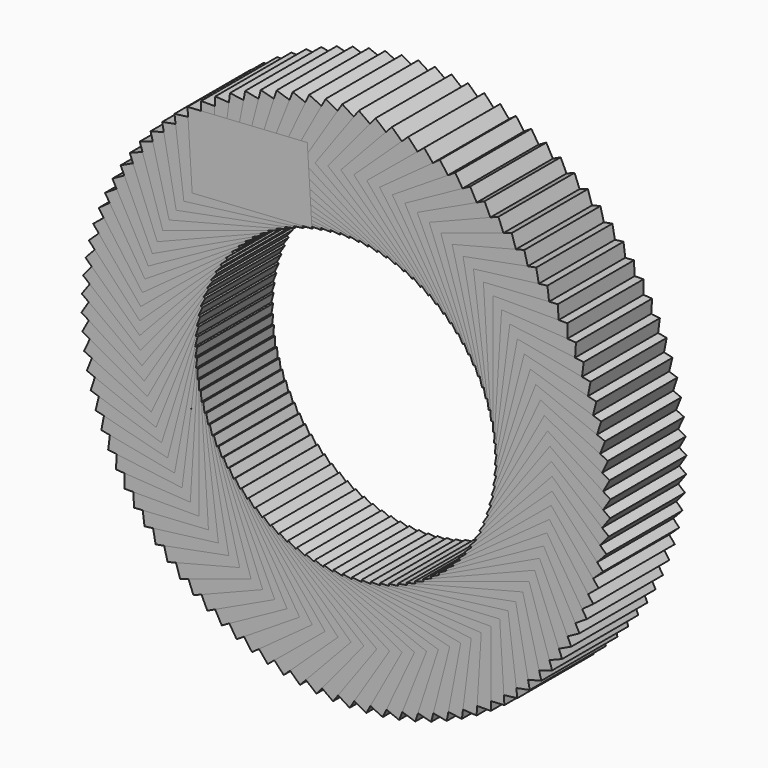
from build123d import *

# Parameters (mm, degrees)
F0_W            = 95.955953002
F0_H            = 59.5492273569
F1_DEPTH        = 76.0588273406
F1_COPIES_COUNT = 100


# Not quite as in the source:
# - a feature of the source that left no trace in its solid (it failed there, or was rolled back) is left out
# - a pattern or mirror of a feature is missing from the dataset's text; its kind, count and spacing are read off the source's solid
# - the program builds the solid bodies; features that only make, move or delete a surface that nothing else refers to are left out


with BuildPart() as f1:
    # F0 (on Front) → F1 (new body)
    with BuildSketch(Plane.XZ):
        with Locations((-90.7992497087, 42.9625064135)):
            Rectangle(F0_W, F0_H)
    extrude(amount=F1_DEPTH)


with BuildPart() as f1_copies_1:
    # F1_copies: instance of F1
    add(f1.part.rotate(Axis((-23.007184, 0, -104.193181), (0, 1, 0)), 1 * 360 / F1_COPIES_COUNT))


with BuildPart() as f1_copies_2:
    # F1_copies: instance of F1
    add(f1.part.rotate(Axis((-23.007184, 0, -104.193181), (0, 1, 0)), 2 * 360 / F1_COPIES_COUNT))


with BuildPart() as f1_copies_3:
    # F1_copies: instance of F1
    add(f1.part.rotate(Axis((-23.007184, 0, -104.193181), (0, 1, 0)), 3 * 360 / F1_COPIES_COUNT))


with BuildPart() as f1_copies_4:
    # F1_copies: instance of F1
    add(f1.part.rotate(Axis((-23.007184, 0, -104.193181), (0, 1, 0)), 4 * 360 / F1_COPIES_COUNT))


with BuildPart() as f1_copies_5:
    # F1_copies: instance of F1
    add(f1.part.rotate(Axis((-23.007184, 0, -104.193181), (0, 1, 0)), 5 * 360 / F1_COPIES_COUNT))


with BuildPart() as f1_copies_6:
    # F1_copies: instance of F1
    add(f1.part.rotate(Axis((-23.007184, 0, -104.193181), (0, 1, 0)), 6 * 360 / F1_COPIES_COUNT))


with BuildPart() as f1_copies_7:
    # F1_copies: instance of F1
    add(f1.part.rotate(Axis((-23.007184, 0, -104.193181), (0, 1, 0)), 7 * 360 / F1_COPIES_COUNT))


with BuildPart() as f1_copies_8:
    # F1_copies: instance of F1
    add(f1.part.rotate(Axis((-23.007184, 0, -104.193181), (0, 1, 0)), 8 * 360 / F1_COPIES_COUNT))


with BuildPart() as f1_copies_9:
    # F1_copies: instance of F1
    add(f1.part.rotate(Axis((-23.007184, 0, -104.193181), (0, 1, 0)), 9 * 360 / F1_COPIES_COUNT))


with BuildPart() as f1_copies_10:
    # F1_copies: instance of F1
    add(f1.part.rotate(Axis((-23.007184, 0, -104.193181), (0, 1, 0)), 10 * 360 / F1_COPIES_COUNT))


with BuildPart() as f1_copies_11:
    # F1_copies: instance of F1
    add(f1.part.rotate(Axis((-23.007184, 0, -104.193181), (0, 1, 0)), 11 * 360 / F1_COPIES_COUNT))


with BuildPart() as f1_copies_12:
    # F1_copies: instance of F1
    add(f1.part.rotate(Axis((-23.007184, 0, -104.193181), (0, 1, 0)), 12 * 360 / F1_COPIES_COUNT))


with BuildPart() as f1_copies_13:
    # F1_copies: instance of F1
    add(f1.part.rotate(Axis((-23.007184, 0, -104.193181), (0, 1, 0)), 13 * 360 / F1_COPIES_COUNT))


with BuildPart() as f1_copies_14:
    # F1_copies: instance of F1
    add(f1.part.rotate(Axis((-23.007184, 0, -104.193181), (0, 1, 0)), 14 * 360 / F1_COPIES_COUNT))


with BuildPart() as f1_copies_15:
    # F1_copies: instance of F1
    add(f1.part.rotate(Axis((-23.007184, 0, -104.193181), (0, 1, 0)), 15 * 360 / F1_COPIES_COUNT))


with BuildPart() as f1_copies_16:
    # F1_copies: instance of F1
    add(f1.part.rotate(Axis((-23.007184, 0, -104.193181), (0, 1, 0)), 16 * 360 / F1_COPIES_COUNT))


with BuildPart() as f1_copies_17:
    # F1_copies: instance of F1
    add(f1.part.rotate(Axis((-23.007184, 0, -104.193181), (0, 1, 0)), 17 * 360 / F1_COPIES_COUNT))


with BuildPart() as f1_copies_18:
    # F1_copies: instance of F1
    add(f1.part.rotate(Axis((-23.007184, 0, -104.193181), (0, 1, 0)), 18 * 360 / F1_COPIES_COUNT))


with BuildPart() as f1_copies_19:
    # F1_copies: instance of F1
    add(f1.part.rotate(Axis((-23.007184, 0, -104.193181), (0, 1, 0)), 19 * 360 / F1_COPIES_COUNT))


with BuildPart() as f1_copies_20:
    # F1_copies: instance of F1
    add(f1.part.rotate(Axis((-23.007184, 0, -104.193181), (0, 1, 0)), 20 * 360 / F1_COPIES_COUNT))


with BuildPart() as f1_copies_21:
    # F1_copies: instance of F1
    add(f1.part.rotate(Axis((-23.007184, 0, -104.193181), (0, 1, 0)), 21 * 360 / F1_COPIES_COUNT))


with BuildPart() as f1_copies_22:
    # F1_copies: instance of F1
    add(f1.part.rotate(Axis((-23.007184, 0, -104.193181), (0, 1, 0)), 22 * 360 / F1_COPIES_COUNT))


with BuildPart() as f1_copies_23:
    # F1_copies: instance of F1
    add(f1.part.rotate(Axis((-23.007184, 0, -104.193181), (0, 1, 0)), 23 * 360 / F1_COPIES_COUNT))


with BuildPart() as f1_copies_24:
    # F1_copies: instance of F1
    add(f1.part.rotate(Axis((-23.007184, 0, -104.193181), (0, 1, 0)), 24 * 360 / F1_COPIES_COUNT))


with BuildPart() as f1_copies_25:
    # F1_copies: instance of F1
    add(f1.part.rotate(Axis((-23.007184, 0, -104.193181), (0, 1, 0)), 25 * 360 / F1_COPIES_COUNT))


with BuildPart() as f1_copies_26:
    # F1_copies: instance of F1
    add(f1.part.rotate(Axis((-23.007184, 0, -104.193181), (0, 1, 0)), 26 * 360 / F1_COPIES_COUNT))


with BuildPart() as f1_copies_27:
    # F1_copies: instance of F1
    add(f1.part.rotate(Axis((-23.007184, 0, -104.193181), (0, 1, 0)), 27 * 360 / F1_COPIES_COUNT))


with BuildPart() as f1_copies_28:
    # F1_copies: instance of F1
    add(f1.part.rotate(Axis((-23.007184, 0, -104.193181), (0, 1, 0)), 28 * 360 / F1_COPIES_COUNT))


with BuildPart() as f1_copies_29:
    # F1_copies: instance of F1
    add(f1.part.rotate(Axis((-23.007184, 0, -104.193181), (0, 1, 0)), 29 * 360 / F1_COPIES_COUNT))


with BuildPart() as f1_copies_30:
    # F1_copies: instance of F1
    add(f1.part.rotate(Axis((-23.007184, 0, -104.193181), (0, 1, 0)), 30 * 360 / F1_COPIES_COUNT))


with BuildPart() as f1_copies_31:
    # F1_copies: instance of F1
    add(f1.part.rotate(Axis((-23.007184, 0, -104.193181), (0, 1, 0)), 31 * 360 / F1_COPIES_COUNT))


with BuildPart() as f1_copies_32:
    # F1_copies: instance of F1
    add(f1.part.rotate(Axis((-23.007184, 0, -104.193181), (0, 1, 0)), 32 * 360 / F1_COPIES_COUNT))


with BuildPart() as f1_copies_33:
    # F1_copies: instance of F1
    add(f1.part.rotate(Axis((-23.007184, 0, -104.193181), (0, 1, 0)), 33 * 360 / F1_COPIES_COUNT))


with BuildPart() as f1_copies_34:
    # F1_copies: instance of F1
    add(f1.part.rotate(Axis((-23.007184, 0, -104.193181), (0, 1, 0)), 34 * 360 / F1_COPIES_COUNT))


with BuildPart() as f1_copies_35:
    # F1_copies: instance of F1
    add(f1.part.rotate(Axis((-23.007184, 0, -104.193181), (0, 1, 0)), 35 * 360 / F1_COPIES_COUNT))


with BuildPart() as f1_copies_36:
    # F1_copies: instance of F1
    add(f1.part.rotate(Axis((-23.007184, 0, -104.193181), (0, 1, 0)), 36 * 360 / F1_COPIES_COUNT))


with BuildPart() as f1_copies_37:
    # F1_copies: instance of F1
    add(f1.part.rotate(Axis((-23.007184, 0, -104.193181), (0, 1, 0)), 37 * 360 / F1_COPIES_COUNT))


with BuildPart() as f1_copies_38:
    # F1_copies: instance of F1
    add(f1.part.rotate(Axis((-23.007184, 0, -104.193181), (0, 1, 0)), 38 * 360 / F1_COPIES_COUNT))


with BuildPart() as f1_copies_39:
    # F1_copies: instance of F1
    add(f1.part.rotate(Axis((-23.007184, 0, -104.193181), (0, 1, 0)), 39 * 360 / F1_COPIES_COUNT))


with BuildPart() as f1_copies_40:
    # F1_copies: instance of F1
    add(f1.part.rotate(Axis((-23.007184, 0, -104.193181), (0, 1, 0)), 40 * 360 / F1_COPIES_COUNT))


with BuildPart() as f1_copies_41:
    # F1_copies: instance of F1
    add(f1.part.rotate(Axis((-23.007184, 0, -104.193181), (0, 1, 0)), 41 * 360 / F1_COPIES_COUNT))


with BuildPart() as f1_copies_42:
    # F1_copies: instance of F1
    add(f1.part.rotate(Axis((-23.007184, 0, -104.193181), (0, 1, 0)), 42 * 360 / F1_COPIES_COUNT))


with BuildPart() as f1_copies_43:
    # F1_copies: instance of F1
    add(f1.part.rotate(Axis((-23.007184, 0, -104.193181), (0, 1, 0)), 43 * 360 / F1_COPIES_COUNT))


with BuildPart() as f1_copies_44:
    # F1_copies: instance of F1
    add(f1.part.rotate(Axis((-23.007184, 0, -104.193181), (0, 1, 0)), 44 * 360 / F1_COPIES_COUNT))


with BuildPart() as f1_copies_45:
    # F1_copies: instance of F1
    add(f1.part.rotate(Axis((-23.007184, 0, -104.193181), (0, 1, 0)), 45 * 360 / F1_COPIES_COUNT))


with BuildPart() as f1_copies_46:
    # F1_copies: instance of F1
    add(f1.part.rotate(Axis((-23.007184, 0, -104.193181), (0, 1, 0)), 46 * 360 / F1_COPIES_COUNT))


with BuildPart() as f1_copies_47:
    # F1_copies: instance of F1
    add(f1.part.rotate(Axis((-23.007184, 0, -104.193181), (0, 1, 0)), 47 * 360 / F1_COPIES_COUNT))


with BuildPart() as f1_copies_48:
    # F1_copies: instance of F1
    add(f1.part.rotate(Axis((-23.007184, 0, -104.193181), (0, 1, 0)), 48 * 360 / F1_COPIES_COUNT))


with BuildPart() as f1_copies_49:
    # F1_copies: instance of F1
    add(f1.part.rotate(Axis((-23.007184, 0, -104.193181), (0, 1, 0)), 49 * 360 / F1_COPIES_COUNT))


with BuildPart() as f1_copies_50:
    # F1_copies: instance of F1
    add(f1.part.rotate(Axis((-23.007184, 0, -104.193181), (0, 1, 0)), 50 * 360 / F1_COPIES_COUNT))


with BuildPart() as f1_copies_51:
    # F1_copies: instance of F1
    add(f1.part.rotate(Axis((-23.007184, 0, -104.193181), (0, 1, 0)), 51 * 360 / F1_COPIES_COUNT))


with BuildPart() as f1_copies_52:
    # F1_copies: instance of F1
    add(f1.part.rotate(Axis((-23.007184, 0, -104.193181), (0, 1, 0)), 52 * 360 / F1_COPIES_COUNT))


with BuildPart() as f1_copies_53:
    # F1_copies: instance of F1
    add(f1.part.rotate(Axis((-23.007184, 0, -104.193181), (0, 1, 0)), 53 * 360 / F1_COPIES_COUNT))


with BuildPart() as f1_copies_54:
    # F1_copies: instance of F1
    add(f1.part.rotate(Axis((-23.007184, 0, -104.193181), (0, 1, 0)), 54 * 360 / F1_COPIES_COUNT))


with BuildPart() as f1_copies_55:
    # F1_copies: instance of F1
    add(f1.part.rotate(Axis((-23.007184, 0, -104.193181), (0, 1, 0)), 55 * 360 / F1_COPIES_COUNT))


with BuildPart() as f1_copies_56:
    # F1_copies: instance of F1
    add(f1.part.rotate(Axis((-23.007184, 0, -104.193181), (0, 1, 0)), 56 * 360 / F1_COPIES_COUNT))


with BuildPart() as f1_copies_57:
    # F1_copies: instance of F1
    add(f1.part.rotate(Axis((-23.007184, 0, -104.193181), (0, 1, 0)), 57 * 360 / F1_COPIES_COUNT))


with BuildPart() as f1_copies_58:
    # F1_copies: instance of F1
    add(f1.part.rotate(Axis((-23.007184, 0, -104.193181), (0, 1, 0)), 58 * 360 / F1_COPIES_COUNT))


with BuildPart() as f1_copies_59:
    # F1_copies: instance of F1
    add(f1.part.rotate(Axis((-23.007184, 0, -104.193181), (0, 1, 0)), 59 * 360 / F1_COPIES_COUNT))


with BuildPart() as f1_copies_60:
    # F1_copies: instance of F1
    add(f1.part.rotate(Axis((-23.007184, 0, -104.193181), (0, 1, 0)), 60 * 360 / F1_COPIES_COUNT))


with BuildPart() as f1_copies_61:
    # F1_copies: instance of F1
    add(f1.part.rotate(Axis((-23.007184, 0, -104.193181), (0, 1, 0)), 61 * 360 / F1_COPIES_COUNT))


with BuildPart() as f1_copies_62:
    # F1_copies: instance of F1
    add(f1.part.rotate(Axis((-23.007184, 0, -104.193181), (0, 1, 0)), 62 * 360 / F1_COPIES_COUNT))


with BuildPart() as f1_copies_63:
    # F1_copies: instance of F1
    add(f1.part.rotate(Axis((-23.007184, 0, -104.193181), (0, 1, 0)), 63 * 360 / F1_COPIES_COUNT))


with BuildPart() as f1_copies_64:
    # F1_copies: instance of F1
    add(f1.part.rotate(Axis((-23.007184, 0, -104.193181), (0, 1, 0)), 64 * 360 / F1_COPIES_COUNT))


with BuildPart() as f1_copies_65:
    # F1_copies: instance of F1
    add(f1.part.rotate(Axis((-23.007184, 0, -104.193181), (0, 1, 0)), 65 * 360 / F1_COPIES_COUNT))


with BuildPart() as f1_copies_66:
    # F1_copies: instance of F1
    add(f1.part.rotate(Axis((-23.007184, 0, -104.193181), (0, 1, 0)), 66 * 360 / F1_COPIES_COUNT))


with BuildPart() as f1_copies_67:
    # F1_copies: instance of F1
    add(f1.part.rotate(Axis((-23.007184, 0, -104.193181), (0, 1, 0)), 67 * 360 / F1_COPIES_COUNT))


with BuildPart() as f1_copies_68:
    # F1_copies: instance of F1
    add(f1.part.rotate(Axis((-23.007184, 0, -104.193181), (0, 1, 0)), 68 * 360 / F1_COPIES_COUNT))


with BuildPart() as f1_copies_69:
    # F1_copies: instance of F1
    add(f1.part.rotate(Axis((-23.007184, 0, -104.193181), (0, 1, 0)), 69 * 360 / F1_COPIES_COUNT))


with BuildPart() as f1_copies_70:
    # F1_copies: instance of F1
    add(f1.part.rotate(Axis((-23.007184, 0, -104.193181), (0, 1, 0)), 70 * 360 / F1_COPIES_COUNT))


with BuildPart() as f1_copies_71:
    # F1_copies: instance of F1
    add(f1.part.rotate(Axis((-23.007184, 0, -104.193181), (0, 1, 0)), 71 * 360 / F1_COPIES_COUNT))


with BuildPart() as f1_copies_72:
    # F1_copies: instance of F1
    add(f1.part.rotate(Axis((-23.007184, 0, -104.193181), (0, 1, 0)), 72 * 360 / F1_COPIES_COUNT))


with BuildPart() as f1_copies_73:
    # F1_copies: instance of F1
    add(f1.part.rotate(Axis((-23.007184, 0, -104.193181), (0, 1, 0)), 73 * 360 / F1_COPIES_COUNT))


with BuildPart() as f1_copies_74:
    # F1_copies: instance of F1
    add(f1.part.rotate(Axis((-23.007184, 0, -104.193181), (0, 1, 0)), 74 * 360 / F1_COPIES_COUNT))


with BuildPart() as f1_copies_75:
    # F1_copies: instance of F1
    add(f1.part.rotate(Axis((-23.007184, 0, -104.193181), (0, 1, 0)), 75 * 360 / F1_COPIES_COUNT))


with BuildPart() as f1_copies_76:
    # F1_copies: instance of F1
    add(f1.part.rotate(Axis((-23.007184, 0, -104.193181), (0, 1, 0)), 76 * 360 / F1_COPIES_COUNT))


with BuildPart() as f1_copies_77:
    # F1_copies: instance of F1
    add(f1.part.rotate(Axis((-23.007184, 0, -104.193181), (0, 1, 0)), 77 * 360 / F1_COPIES_COUNT))


with BuildPart() as f1_copies_78:
    # F1_copies: instance of F1
    add(f1.part.rotate(Axis((-23.007184, 0, -104.193181), (0, 1, 0)), 78 * 360 / F1_COPIES_COUNT))


with BuildPart() as f1_copies_79:
    # F1_copies: instance of F1
    add(f1.part.rotate(Axis((-23.007184, 0, -104.193181), (0, 1, 0)), 79 * 360 / F1_COPIES_COUNT))


with BuildPart() as f1_copies_80:
    # F1_copies: instance of F1
    add(f1.part.rotate(Axis((-23.007184, 0, -104.193181), (0, 1, 0)), 80 * 360 / F1_COPIES_COUNT))


with BuildPart() as f1_copies_81:
    # F1_copies: instance of F1
    add(f1.part.rotate(Axis((-23.007184, 0, -104.193181), (0, 1, 0)), 81 * 360 / F1_COPIES_COUNT))


with BuildPart() as f1_copies_82:
    # F1_copies: instance of F1
    add(f1.part.rotate(Axis((-23.007184, 0, -104.193181), (0, 1, 0)), 82 * 360 / F1_COPIES_COUNT))


with BuildPart() as f1_copies_83:
    # F1_copies: instance of F1
    add(f1.part.rotate(Axis((-23.007184, 0, -104.193181), (0, 1, 0)), 83 * 360 / F1_COPIES_COUNT))


with BuildPart() as f1_copies_84:
    # F1_copies: instance of F1
    add(f1.part.rotate(Axis((-23.007184, 0, -104.193181), (0, 1, 0)), 84 * 360 / F1_COPIES_COUNT))


with BuildPart() as f1_copies_85:
    # F1_copies: instance of F1
    add(f1.part.rotate(Axis((-23.007184, 0, -104.193181), (0, 1, 0)), 85 * 360 / F1_COPIES_COUNT))


with BuildPart() as f1_copies_86:
    # F1_copies: instance of F1
    add(f1.part.rotate(Axis((-23.007184, 0, -104.193181), (0, 1, 0)), 86 * 360 / F1_COPIES_COUNT))


with BuildPart() as f1_copies_87:
    # F1_copies: instance of F1
    add(f1.part.rotate(Axis((-23.007184, 0, -104.193181), (0, 1, 0)), 87 * 360 / F1_COPIES_COUNT))


with BuildPart() as f1_copies_88:
    # F1_copies: instance of F1
    add(f1.part.rotate(Axis((-23.007184, 0, -104.193181), (0, 1, 0)), 88 * 360 / F1_COPIES_COUNT))


with BuildPart() as f1_copies_89:
    # F1_copies: instance of F1
    add(f1.part.rotate(Axis((-23.007184, 0, -104.193181), (0, 1, 0)), 89 * 360 / F1_COPIES_COUNT))


with BuildPart() as f1_copies_90:
    # F1_copies: instance of F1
    add(f1.part.rotate(Axis((-23.007184, 0, -104.193181), (0, 1, 0)), 90 * 360 / F1_COPIES_COUNT))


with BuildPart() as f1_copies_91:
    # F1_copies: instance of F1
    add(f1.part.rotate(Axis((-23.007184, 0, -104.193181), (0, 1, 0)), 91 * 360 / F1_COPIES_COUNT))


with BuildPart() as f1_copies_92:
    # F1_copies: instance of F1
    add(f1.part.rotate(Axis((-23.007184, 0, -104.193181), (0, 1, 0)), 92 * 360 / F1_COPIES_COUNT))


with BuildPart() as f1_copies_93:
    # F1_copies: instance of F1
    add(f1.part.rotate(Axis((-23.007184, 0, -104.193181), (0, 1, 0)), 93 * 360 / F1_COPIES_COUNT))


with BuildPart() as f1_copies_94:
    # F1_copies: instance of F1
    add(f1.part.rotate(Axis((-23.007184, 0, -104.193181), (0, 1, 0)), 94 * 360 / F1_COPIES_COUNT))


with BuildPart() as f1_copies_95:
    # F1_copies: instance of F1
    add(f1.part.rotate(Axis((-23.007184, 0, -104.193181), (0, 1, 0)), 95 * 360 / F1_COPIES_COUNT))


with BuildPart() as f1_copies_96:
    # F1_copies: instance of F1
    add(f1.part.rotate(Axis((-23.007184, 0, -104.193181), (0, 1, 0)), 96 * 360 / F1_COPIES_COUNT))


with BuildPart() as f1_copies_97:
    # F1_copies: instance of F1
    add(f1.part.rotate(Axis((-23.007184, 0, -104.193181), (0, 1, 0)), 97 * 360 / F1_COPIES_COUNT))


with BuildPart() as f1_copies_98:
    # F1_copies: instance of F1
    add(f1.part.rotate(Axis((-23.007184, 0, -104.193181), (0, 1, 0)), 98 * 360 / F1_COPIES_COUNT))


with BuildPart() as f1_copies_99:
    # F1_copies: instance of F1
    add(f1.part.rotate(Axis((-23.007184, 0, -104.193181), (0, 1, 0)), 99 * 360 / F1_COPIES_COUNT))


solid = Compound([f1.part, f1_copies_1.part, f1_copies_2.part, f1_copies_3.part, f1_copies_4.part, f1_copies_5.part, f1_copies_6.part, f1_copies_7.part, f1_copies_8.part, f1_copies_9.part, f1_copies_10.part, f1_copies_11.part, f1_copies_12.part, f1_copies_13.part, f1_copies_14.part, f1_copies_15.part, f1_copies_16.part, f1_copies_17.part, f1_copies_18.part, f1_copies_19.part, f1_copies_20.part, f1_copies_21.part, f1_copies_22.part, f1_copies_23.part, f1_copies_24.part, f1_copies_25.part, f1_copies_26.part, f1_copies_27.part, f1_copies_28.part, f1_copies_29.part, f1_copies_30.part, f1_copies_31.part, f1_copies_32.part, f1_copies_33.part, f1_copies_34.part, f1_copies_35.part, f1_copies_36.part, f1_copies_37.part, f1_copies_38.part, f1_copies_39.part, f1_copies_40.part, f1_copies_41.part, f1_copies_42.part, f1_copies_43.part, f1_copies_44.part, f1_copies_45.part, f1_copies_46.part, f1_copies_47.part, f1_copies_48.part, f1_copies_49.part, f1_copies_50.part, f1_copies_51.part, f1_copies_52.part, f1_copies_53.part, f1_copies_54.part, f1_copies_55.part, f1_copies_56.part, f1_copies_57.part, f1_copies_58.part, f1_copies_59.part, f1_copies_60.part, f1_copies_61.part, f1_copies_62.part, f1_copies_63.part, f1_copies_64.part, f1_copies_65.part, f1_copies_66.part, f1_copies_67.part, f1_copies_68.part, f1_copies_69.part, f1_copies_70.part, f1_copies_71.part, f1_copies_72.part, f1_copies_73.part, f1_copies_74.part, f1_copies_75.part, f1_copies_76.part, f1_copies_77.part, f1_copies_78.part, f1_copies_79.part, f1_copies_80.part, f1_copies_81.part, f1_copies_82.part, f1_copies_83.part, f1_copies_84.part, f1_copies_85.part, f1_copies_86.part, f1_copies_87.part, f1_copies_88.part, f1_copies_89.part, f1_copies_90.part, f1_copies_91.part, f1_copies_92.part, f1_copies_93.part, f1_copies_94.part, f1_copies_95.part, f1_copies_96.part, f1_copies_97.part, f1_copies_98.part, f1_copies_99.part])
